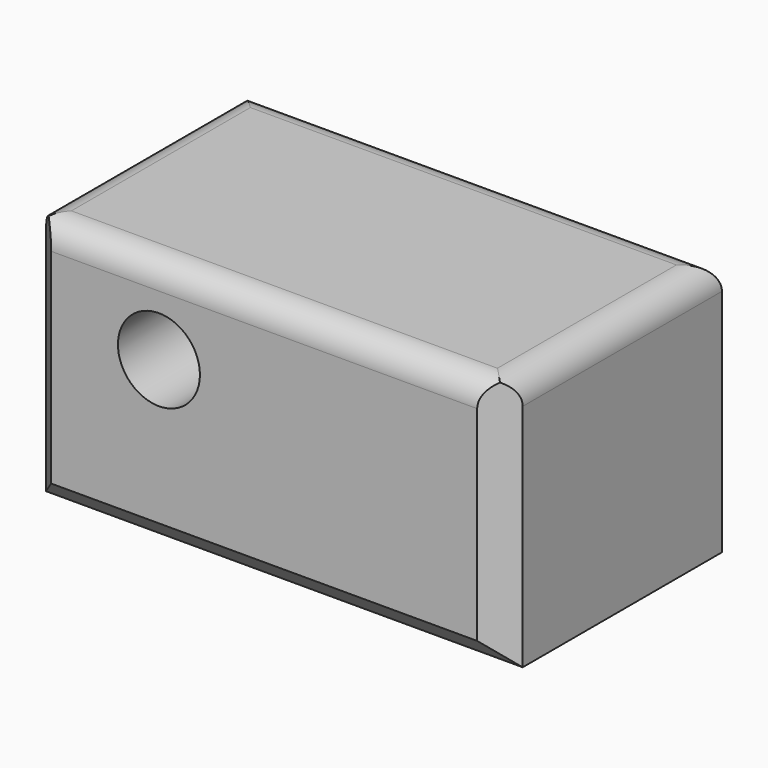
from build123d import *

# Parameters (mm, degrees)
F0_W        = 95.7747641951
F0_H        = 51.2457955629
F1_DEPTH    = 55.118
F2_R        = 5.08
F3_T1_DEPTH = 72.2940947206
F3_T3_DEPTH = 121.9030633528
F4_R        = 8.2354501167
F5_DEPTH    = 129.032


# Not quite as in the source:
# - a fillet or chamfer that OpenCascade refuses, or shapes differently, is made with other operations: its cross-section is extruded or revolved along the edge and cut away or added


with BuildPart() as f1:
    # F0 (on Front) → F1 (new body)
    with BuildSketch(Plane.XZ):
        with Locations((-20.3259242699, 5.727651529)):
            Rectangle(F0_W, F0_H)
    extrude(amount=F1_DEPTH)

    # F2
    f2_edges = [f1.edges().sort_by_distance(p)[0] for p in [
        (27.561458, -27.559, 31.350549),
        (-68.213306, -27.559, 31.350549),
        (-20.325924, 0, 31.350549),
        (-20.325924, -55.118, 31.350549),
    ]]
    fillet(f2_edges, radius=F2_R)

    # F3: chamfer of 5.08 on 4 edges, made by hand

    # F3_s2 → F3_t1 (cut)
    with BuildSketch(Plane.XY.offset(-32.9593958313)):
        Polygon((-63.1333063674, -55.118), (-68.2133063674, -50.038), (-68.2133063674, -55.118), align=None)
        Polygon((27.5614578277, -50.038), (22.4814578277, -55.118), (27.5614578277, -55.118), align=None)
    extrude(amount=F3_T1_DEPTH, mode=Mode.SUBTRACT)

    # F3_s4 → F3_t3 (cut)
    with BuildSketch(Plane.YZ.offset(-81.2774559463)):
        Polygon((-55.118, -14.8152462524), (-50.038, -19.8952462524), (-55.118, -19.8952462524), align=None)
    extrude(amount=F3_T3_DEPTH, mode=Mode.SUBTRACT)

    # F4 (on face) → F5 (cut)
    with BuildSketch(Plane.XZ.offset(55.118)):
        with Locations((-41.4717569947, 14.13862966)):
            Circle(F4_R)
    extrude(amount=-F5_DEPTH, mode=Mode.SUBTRACT)


solid = f1.part
